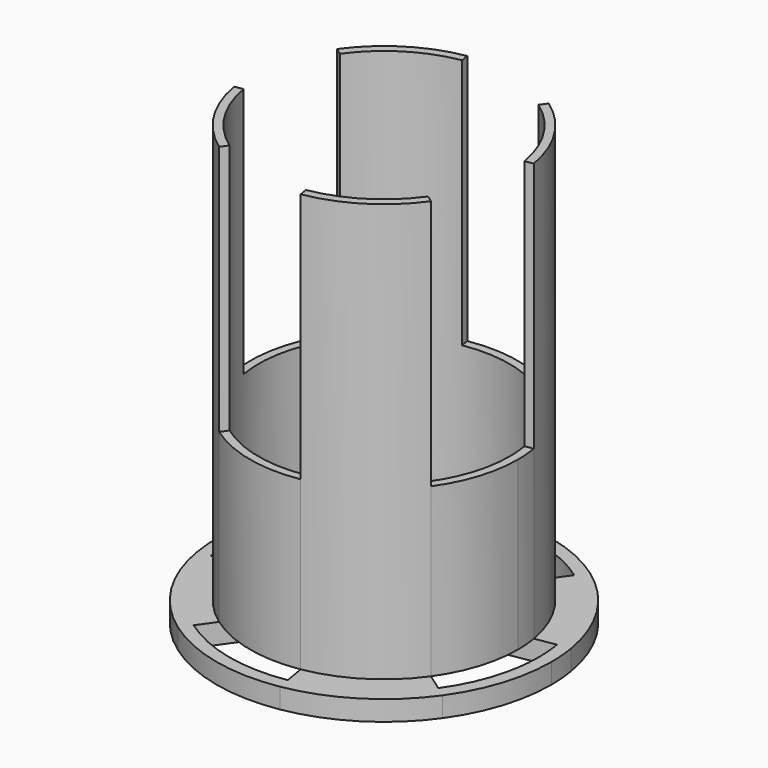
from build123d import *

# Parameters (mm, degrees)
F1_DEPTH = 1.2
F2_DEPTH = 6
F4_DEPTH = 25
F5_DEPTH = 10


with BuildPart() as f1:
    # F0 (on Top) → F1 (new body)
    with BuildSketch(Plane.XY):
        with BuildLine():
            ThreePointArc((8.1482783535, -5.7970302633), (9.5258276159, -3.0427961207), (10, 0))
            ThreePointArc((10, 0), (9.965144828, 0.8341993506), (9.8608222887, 1.6625834689))
            Line((9.8608222887, 1.6625834689), (9.0045502887, -2.0672235383))
            Line((9.0045502887, -2.0672235383), (8.1482783535, -5.7970302633))
        make_face()
        with BuildLine():
            Line((7.8289263433, 4.9054308037), (9.8608222887, 1.6625834689))
            ThreePointArc((9.8608222887, 1.6625834689), (8.4739687378, 5.3096001573), (5.7970302633, 8.1482783535))
            Line((5.7970302633, 8.1482783535), (7.8289263433, 4.9054308037))
        make_face()
        with BuildLine():
            Line((9.1102118863, 1.536026838), (9.8608222887, 1.6625834689))
            Line((9.8608222887, 1.6625834689), (7.8289263433, 4.9054308037))
            ThreePointArc((7.8289263433, 4.9054308037), (8.6354977715, 3.2838266242), (9.1102118863, 1.536026838))
        make_face()
        with BuildLine():
            Line((9.0045502887, -2.0672235383), (9.8608222887, 1.6625834689))
            Line((9.8608222887, 1.6625834689), (9.1102118863, 1.536026838))
            ThreePointArc((9.1102118863, 1.536026838), (9.2065933451, 0.7706997061), (9.2387953251, 0))
            ThreePointArc((9.2387953251, 0), (9.1800472812, -1.040226405), (9.0045502887, -2.0672235383))
        make_face()
        with BuildLine():
            Line((7.528027596, -5.3557576096), (8.1482783535, -5.7970302633))
            Line((8.1482783535, -5.7970302633), (9.0045502887, -2.0672235383))
            ThreePointArc((9.0045502887, -2.0672235383), (8.4282351037, -3.7842029671), (7.528027596, -5.3557576096))
        make_face()
        with BuildLine():
            ThreePointArc((1.6625834689, -9.8608222887), (5.3096001573, -8.4739687378), (8.1482783535, -5.7970302633))
            Line((8.1482783535, -5.7970302633), (4.9054307168, -7.8289263978))
            Line((4.9054307168, -7.8289263978), (1.6625834689, -9.8608222887))
        make_face()
        with BuildLine():
            Line((4.9054307168, -7.8289263978), (8.1482783535, -5.7970302633))
            Line((8.1482783535, -5.7970302633), (7.528027596, -5.3557576096))
            ThreePointArc((7.528027596, -5.3557576096), (6.3385220965, -6.7214936355), (4.9054307168, -7.8289263978))
        make_face()
        with BuildLine():
            Line((2.0672236693, 9.0045502586), (5.7970302633, 8.1482783535))
            ThreePointArc((5.7970302633, 8.1482783535), (2.2375464814, 9.7464550347), (-1.6625834689, 9.8608222887))
            Line((-1.6625834689, 9.8608222887), (2.0672236693, 9.0045502586))
        make_face()
        with BuildLine():
            Line((5.3557576096, 7.528027596), (5.7970302633, 8.1482783535))
            Line((5.7970302633, 8.1482783535), (2.0672236693, 9.0045502586))
            ThreePointArc((2.0672236693, 9.0045502586), (3.7842030284, 8.4282350762), (5.3557576096, 7.528027596))
        make_face()
        with BuildLine():
            Line((7.8289263433, 4.9054308037), (5.7970302633, 8.1482783535))
            Line((5.7970302633, 8.1482783535), (5.3557576096, 7.528027596))
            ThreePointArc((5.3557576096, 7.528027596), (6.7214936003, 6.3385221338), (7.8289263433, 4.9054308037))
        make_face()
        with BuildLine():
            Line((1.536026838, -9.1102118863), (1.6625834689, -9.8608222887))
            Line((1.6625834689, -9.8608222887), (4.9054307168, -7.8289263978))
            ThreePointArc((4.9054307168, -7.8289263978), (3.2838265763, -8.6354977897), (1.536026838, -9.1102118863))
        make_face()
        with BuildLine():
            ThreePointArc((-5.7970302633, -8.1482783535), (-2.2375464814, -9.7464550347), (1.6625834689, -9.8608222887))
            Line((1.6625834689, -9.8608222887), (-2.0672231954, -9.0045503674))
            Line((-2.0672231954, -9.0045503674), (-5.7970302633, -8.1482783535))
        make_face()
        with BuildLine():
            Line((-2.0672231954, -9.0045503674), (1.6625834689, -9.8608222887))
            Line((1.6625834689, -9.8608222887), (1.536026838, -9.1102118863))
            ThreePointArc((1.536026838, -9.1102118863), (-0.2708015541, -9.2348256929), (-2.0672231954, -9.0045503674))
        make_face()
        with BuildLine():
            Line((-4.9054310148, 7.828926211), (-1.6625834689, 9.8608222887))
            ThreePointArc((-1.6625834689, 9.8608222887), (-5.3096001573, 8.4739687378), (-8.1482783535, 5.7970302633))
            Line((-8.1482783535, 5.7970302633), (-4.9054310148, 7.828926211))
        make_face()
        with BuildLine():
            Line((-1.536026838, 9.1102118863), (-1.6625834689, 9.8608222887))
            Line((-1.6625834689, 9.8608222887), (-4.9054310148, 7.828926211))
            ThreePointArc((-4.9054310148, 7.828926211), (-3.2838267407, 8.6354977272), (-1.536026838, 9.1102118863))
        make_face()
        with BuildLine():
            Line((2.0672236693, 9.0045502586), (-1.6625834689, 9.8608222887))
            Line((-1.6625834689, 9.8608222887), (-1.536026838, 9.1102118863))
            ThreePointArc((-1.536026838, 9.1102118863), (0.2708017971, 9.2348256857), (2.0672236693, 9.0045502586))
        make_face()
        with BuildLine():
            Line((-5.3557576096, -7.528027596), (-5.7970302633, -8.1482783535))
            Line((-5.7970302633, -8.1482783535), (-2.0672231954, -9.0045503674))
            ThreePointArc((-2.0672231954, -9.0045503674), (-3.7842028066, -8.4282351757), (-5.3557576096, -7.528027596))
        make_face()
        with BuildLine():
            ThreePointArc((-9.8608222887, -1.6625834689), (-8.4739687378, -5.3096001573), (-5.7970302633, -8.1482783535))
            Line((-5.7970302633, -8.1482783535), (-7.8289263978, -4.9054307168))
            Line((-7.8289263978, -4.9054307168), (-9.8608222887, -1.6625834689))
        make_face()
        with BuildLine():
            Line((-7.8289263978, -4.9054307168), (-5.7970302633, -8.1482783535))
            Line((-5.7970302633, -8.1482783535), (-5.3557576096, -7.528027596))
            ThreePointArc((-5.3557576096, -7.528027596), (-6.7214936355, -6.3385220965), (-7.8289263978, -4.9054307168))
        make_face()
        with BuildLine():
            Line((-9.004550337, 2.0672233281), (-8.1482783535, 5.7970302633))
            ThreePointArc((-8.1482783535, 5.7970302633), (-9.7464550347, 2.2375464814), (-9.8608222887, -1.6625834689))
            Line((-9.8608222887, -1.6625834689), (-9.004550337, 2.0672233281))
        make_face()
        with BuildLine():
            Line((-7.528027596, 5.3557576096), (-8.1482783535, 5.7970302633))
            Line((-8.1482783535, 5.7970302633), (-9.004550337, 2.0672233281))
            ThreePointArc((-9.004550337, 2.0672233281), (-8.4282351479, 3.7842028687), (-7.528027596, 5.3557576096))
        make_face()
        with BuildLine():
            Line((-4.9054310148, 7.828926211), (-8.1482783535, 5.7970302633))
            Line((-8.1482783535, 5.7970302633), (-7.528027596, 5.3557576096))
            ThreePointArc((-7.528027596, 5.3557576096), (-6.3385222244, 6.7214935148), (-4.9054310148, 7.828926211))
        make_face()
        with BuildLine():
            Line((-9.1102118863, -1.536026838), (-9.8608222887, -1.6625834689))
            Line((-9.8608222887, -1.6625834689), (-7.8289263978, -4.9054307168))
            ThreePointArc((-7.8289263978, -4.9054307168), (-8.6354977897, -3.2838265763), (-9.1102118863, -1.536026838))
        make_face()
        with BuildLine():
            Line((-9.004550337, 2.0672233281), (-9.8608222887, -1.6625834689))
            Line((-9.8608222887, -1.6625834689), (-9.1102118863, -1.536026838))
            ThreePointArc((-9.1102118863, -1.536026838), (-9.2348256909, 0.2708016221), (-9.004550337, 2.0672233281))
        make_face()
        with BuildLine():
            ThreePointArc((-4.9304111443, -0.8312917344), (-4.2369843689, -2.6548000787), (-2.8985151316, -4.0741391768))
            Line((-2.8985151316, -4.0741391768), (-1.1594060527, -1.6296556707))
            ThreePointArc((-1.1594060527, -1.6296556707), (-1.6947937476, -1.0619200315), (-1.9721644577, -0.3325166938))
            Line((-1.9721644577, -0.3325166938), (-4.9304111443, -0.8312917344))
        make_face()
        with BuildLine():
            Line((-1.6296556707, 1.1594060527), (-4.0741391768, 2.8985151316))
            ThreePointArc((-4.0741391768, 2.8985151316), (-4.8732275174, 1.1187732407), (-4.9304111443, -0.8312917344))
            Line((-4.9304111443, -0.8312917344), (-1.9721644577, -0.3325166938))
            ThreePointArc((-1.9721644577, -0.3325166938), (-1.9492910069, 0.4475092963), (-1.6296556707, 1.1594060527))
        make_face()
        with BuildLine():
            Line((-0.3325166938, 1.9721644577), (-0.8312917344, 4.9304111443))
            ThreePointArc((-0.8312917344, 4.9304111443), (-2.6548000787, 4.2369843689), (-4.0741391768, 2.8985151316))
            Line((-4.0741391768, 2.8985151316), (-1.6296556707, 1.1594060527))
            ThreePointArc((-1.6296556707, 1.1594060527), (-1.0619200315, 1.6947937476), (-0.3325166938, 1.9721644577))
        make_face()
        with BuildLine():
            Line((1.1594060527, 1.6296556707), (2.8985151316, 4.0741391768))
            ThreePointArc((2.8985151316, 4.0741391768), (1.1187732407, 4.8732275174), (-0.8312917344, 4.9304111443))
            Line((-0.8312917344, 4.9304111443), (-0.3325166938, 1.9721644577))
            ThreePointArc((-0.3325166938, 1.9721644577), (0.4475092963, 1.9492910069), (1.1594060527, 1.6296556707))
        make_face()
        with BuildLine():
            Line((1.9721644577, 0.3325166938), (4.9304111443, 0.8312917344))
            ThreePointArc((4.9304111443, 0.8312917344), (4.2369843689, 2.6548000787), (2.8985151316, 4.0741391768))
            Line((2.8985151316, 4.0741391768), (1.1594060527, 1.6296556707))
            ThreePointArc((1.1594060527, 1.6296556707), (1.6947937476, 1.0619200315), (1.9721644577, 0.3325166938))
        make_face()
        with BuildLine():
            ThreePointArc((5, 0), (4.982572414, 0.4170996753), (4.9304111443, 0.8312917344))
            Line((4.9304111443, 0.8312917344), (1.9721644577, 0.3325166938))
            ThreePointArc((1.9721644577, 0.3325166938), (1.9930289656, 0.1668398701), (2, 0))
            ThreePointArc((2, 0), (1.9051655232, -0.6085592241), (1.6296556707, -1.1594060527))
            Line((1.6296556707, -1.1594060527), (4.0741391768, -2.8985151316))
            ThreePointArc((4.0741391768, -2.8985151316), (4.7629138079, -1.5213980604), (5, 0))
        make_face()
        with BuildLine():
            ThreePointArc((0.8312917344, -4.9304111443), (2.6548000787, -4.2369843689), (4.0741391768, -2.8985151316))
            Line((4.0741391768, -2.8985151316), (1.6296556707, -1.1594060527))
            ThreePointArc((1.6296556707, -1.1594060527), (1.0619200315, -1.6947937476), (0.3325166938, -1.9721644577))
            Line((0.3325166938, -1.9721644577), (0.8312917344, -4.9304111443))
        make_face()
        with BuildLine():
            ThreePointArc((-2.8985151316, -4.0741391768), (-1.1187732407, -4.8732275174), (0.8312917344, -4.9304111443))
            Line((0.8312917344, -4.9304111443), (0.3325166938, -1.9721644577))
            ThreePointArc((0.3325166938, -1.9721644577), (-0.4475092963, -1.9492910069), (-1.1594060527, -1.6296556707))
            Line((-1.1594060527, -1.6296556707), (-2.8985151316, -4.0741391768))
        make_face()
        with BuildLine():
            ThreePointArc((1.536026838, -9.1102118863), (3.2838265763, -8.6354977897), (4.9054307168, -7.8289263978))
            ThreePointArc((4.9054307168, -7.8289263978), (6.3385220965, -6.7214936355), (7.528027596, -5.3557576096))
            Line((7.528027596, -5.3557576096), (4.0741391768, -2.8985151316))
            ThreePointArc((4.0741391768, -2.8985151316), (2.6548000787, -4.2369843689), (0.8312917344, -4.9304111443))
            Line((0.8312917344, -4.9304111443), (1.536026838, -9.1102118863))
        make_face()
        with BuildLine():
            ThreePointArc((9.1102118863, 1.536026838), (8.6354977715, 3.2838266242), (7.8289263433, 4.9054308037))
            ThreePointArc((7.8289263433, 4.9054308037), (6.7214936003, 6.3385221338), (5.3557576096, 7.528027596))
            Line((5.3557576096, 7.528027596), (2.8985151316, 4.0741391768))
            ThreePointArc((2.8985151316, 4.0741391768), (4.2369843689, 2.6548000787), (4.9304111443, 0.8312917344))
            Line((4.9304111443, 0.8312917344), (9.1102118863, 1.536026838))
        make_face()
        with BuildLine():
            ThreePointArc((-1.536026838, 9.1102118863), (-3.2838267407, 8.6354977272), (-4.9054310148, 7.828926211))
            ThreePointArc((-4.9054310148, 7.828926211), (-6.3385222244, 6.7214935148), (-7.528027596, 5.3557576096))
            Line((-7.528027596, 5.3557576096), (-4.0741391768, 2.8985151316))
            ThreePointArc((-4.0741391768, 2.8985151316), (-2.6548000787, 4.2369843689), (-0.8312917344, 4.9304111443))
            Line((-0.8312917344, 4.9304111443), (-1.536026838, 9.1102118863))
        make_face()
        with BuildLine():
            ThreePointArc((-9.1102118863, -1.536026838), (-8.6354977897, -3.2838265763), (-7.8289263978, -4.9054307168))
            ThreePointArc((-7.8289263978, -4.9054307168), (-6.7214936355, -6.3385220965), (-5.3557576096, -7.528027596))
            Line((-5.3557576096, -7.528027596), (-2.8985151316, -4.0741391768))
            ThreePointArc((-2.8985151316, -4.0741391768), (-4.2369843689, -2.6548000787), (-4.9304111443, -0.8312917344))
            Line((-4.9304111443, -0.8312917344), (-9.1102118863, -1.536026838))
        make_face()
    extrude(amount=F1_DEPTH)

    # F0 (on Top) → F2 (join)
    with BuildSketch(Plane.XY):
        with BuildLine():
            Line((-0.1828841816, 1.0846904518), (-0.3325166938, 1.9721644577))
            ThreePointArc((-0.3325166938, 1.9721644577), (-1.0619200315, 1.6947937476), (-1.6296556707, 1.1594060527))
            Line((-1.6296556707, 1.1594060527), (-0.8963106189, 0.637673329))
            ThreePointArc((-0.8963106189, 0.637673329), (-0.5840560173, 0.9321365612), (-0.1828841816, 1.0846904518))
        make_face()
        with BuildLine():
            Line((-0.8963106189, 0.637673329), (-1.6296556707, 1.1594060527))
            ThreePointArc((-1.6296556707, 1.1594060527), (-1.9492910069, 0.4475092963), (-1.9721644577, -0.3325166938))
            Line((-1.9721644577, -0.3325166938), (-1.0846904518, -0.1828841816))
            ThreePointArc((-1.0846904518, -0.1828841816), (-1.0721100538, 0.246130113), (-0.8963106189, 0.637673329))
        make_face()
        with BuildLine():
            ThreePointArc((-1.9721644577, -0.3325166938), (-1.6947937476, -1.0619200315), (-1.1594060527, -1.6296556707))
            Line((-1.1594060527, -1.6296556707), (-0.637673329, -0.8963106189))
            ThreePointArc((-0.637673329, -0.8963106189), (-0.9321365612, -0.5840560173), (-1.0846904518, -0.1828841816))
            Line((-1.0846904518, -0.1828841816), (-1.9721644577, -0.3325166938))
        make_face()
        with BuildLine():
            ThreePointArc((-1.1594060527, -1.6296556707), (-0.4475092963, -1.9492910069), (0.3325166938, -1.9721644577))
            Line((0.3325166938, -1.9721644577), (0.1828841816, -1.0846904518))
            ThreePointArc((0.1828841816, -1.0846904518), (-0.246130113, -1.0721100538), (-0.637673329, -0.8963106189))
            Line((-0.637673329, -0.8963106189), (-1.1594060527, -1.6296556707))
        make_face()
        with BuildLine():
            ThreePointArc((0.3325166938, -1.9721644577), (1.0619200315, -1.6947937476), (1.6296556707, -1.1594060527))
            Line((1.6296556707, -1.1594060527), (0.8963106189, -0.637673329))
            ThreePointArc((0.8963106189, -0.637673329), (0.5840560173, -0.9321365612), (0.1828841816, -1.0846904518))
            Line((0.1828841816, -1.0846904518), (0.3325166938, -1.9721644577))
        make_face()
        with BuildLine():
            ThreePointArc((2, 0), (1.9930289656, 0.1668398701), (1.9721644577, 0.3325166938))
            Line((1.9721644577, 0.3325166938), (1.0846904518, 0.1828841816))
            ThreePointArc((1.0846904518, 0.1828841816), (1.0961659311, 0.0917619286), (1.1, 0))
            ThreePointArc((1.1, 0), (1.0478410377, -0.3347075733), (0.8963106189, -0.637673329))
            Line((0.8963106189, -0.637673329), (1.6296556707, -1.1594060527))
            ThreePointArc((1.6296556707, -1.1594060527), (1.9051655232, -0.6085592241), (2, 0))
        make_face()
        with BuildLine():
            Line((1.0846904518, 0.1828841816), (1.9721644577, 0.3325166938))
            ThreePointArc((1.9721644577, 0.3325166938), (1.6947937476, 1.0619200315), (1.1594060527, 1.6296556707))
            Line((1.1594060527, 1.6296556707), (0.637673329, 0.8963106189))
            ThreePointArc((0.637673329, 0.8963106189), (0.9321365612, 0.5840560173), (1.0846904518, 0.1828841816))
        make_face()
        with BuildLine():
            Line((0.637673329, 0.8963106189), (1.1594060527, 1.6296556707))
            ThreePointArc((1.1594060527, 1.6296556707), (0.4475092963, 1.9492910069), (-0.3325166938, 1.9721644577))
            Line((-0.3325166938, 1.9721644577), (-0.1828841816, 1.0846904518))
            ThreePointArc((-0.1828841816, 1.0846904518), (0.246130113, 1.0721100538), (0.637673329, 0.8963106189))
        make_face()
    extrude(amount=F2_DEPTH)


with BuildPart() as f4:
    # F3 (on face) → F4 (new body)
    with BuildSketch(Plane.XY.offset(1.2)):
        with BuildLine():
            Line((6.5186226828, -4.6376242106), (6.1112087651, -4.3477726975))
            ThreePointArc((6.1112087651, -4.3477726975), (3.982200118, -6.3554765533), (1.2469376016, -7.3956167165))
            Line((1.2469376016, -7.3956167165), (1.3300667751, -7.888657831))
            ThreePointArc((1.3300667751, -7.888657831), (4.2476801259, -6.7791749902), (6.5186226828, -4.6376242106))
        make_face()
    extrude(amount=F4_DEPTH)



with BuildPart() as f4b:
    # F3 (on face) → F4, piece 2 (new body)
    with BuildSketch(Plane.XY.offset(1.2)):
        with BuildLine():
            ThreePointArc((-6.1112087651, 4.3477726975), (-3.982200118, 6.3554765533), (-1.2469376016, 7.3956167165))
            Line((-1.2469376016, 7.3956167165), (-1.3300667751, 7.888657831))
            ThreePointArc((-1.3300667751, 7.888657831), (-4.2476801259, 6.7791749902), (-6.5186226828, 4.6376242106))
            Line((-6.5186226828, 4.6376242106), (-6.1112087651, 4.3477726975))
        make_face()
    extrude(amount=F4_DEPTH)


with BuildPart() as f4c:
    # F3 (on face) → F4, piece 3 (new body)
    with BuildSketch(Plane.XY.offset(1.2)):
        with BuildLine():
            ThreePointArc((4.3477726975, 6.1112087651), (6.3554765533, 3.982200118), (7.3956167165, 1.2469376016))
            Line((7.3956167165, 1.2469376016), (7.888657831, 1.3300667751))
            ThreePointArc((7.888657831, 1.3300667751), (6.7791749902, 4.2476801259), (4.6376242106, 6.5186226828))
            Line((4.6376242106, 6.5186226828), (4.3477726975, 6.1112087651))
        make_face()
    extrude(amount=F4_DEPTH)


with BuildPart() as f4d:
    # F3 (on face) → F4, piece 4 (new body)
    with BuildSketch(Plane.XY.offset(1.2)):
        with BuildLine():
            Line((-4.6376242106, -6.5186226828), (-4.3477726975, -6.1112087651))
            ThreePointArc((-4.3477726975, -6.1112087651), (-6.3554765533, -3.982200118), (-7.3956167165, -1.2469376016))
            Line((-7.3956167165, -1.2469376016), (-7.888657831, -1.3300667751))
            ThreePointArc((-7.888657831, -1.3300667751), (-6.7791749902, -4.2476801259), (-4.6376242106, -6.5186226828))
        make_face()
    extrude(amount=F4_DEPTH)


with BuildPart() as f4_1:
    add(f4.part)

    add(f4b.part)  # F5 merges F4b

    add(f4c.part)  # F5 merges F4c

    add(f4d.part)  # F5 merges F4d
    # F3 (on face) → F5 (join)
    with BuildSketch(Plane.XY.offset(1.2)):
        with BuildLine():
            Line((1.3300667751, -7.888657831), (1.2469376016, -7.3956167165))
            ThreePointArc((1.2469376016, -7.3956167165), (-1.6781598611, -7.309841276), (-4.3477726975, -6.1112087651))
            Line((-4.3477726975, -6.1112087651), (-4.6376242106, -6.5186226828))
            ThreePointArc((-4.6376242106, -6.5186226828), (-1.7900371851, -7.7971640278), (1.3300667751, -7.888657831))
        make_face()
        with BuildLine():
            ThreePointArc((7.3956167165, 1.2469376016), (7.473858621, 0.625649513), (7.5, 0))
            ThreePointArc((7.5, 0), (7.1443707119, -2.2820970906), (6.1112087651, -4.3477726975))
            Line((6.1112087651, -4.3477726975), (6.5186226828, -4.6376242106))
            ThreePointArc((6.5186226828, -4.6376242106), (7.6206620927, -2.4342368966), (8, 0))
            ThreePointArc((8, 0), (7.9721158624, 0.6673594805), (7.888657831, 1.3300667751))
            Line((7.888657831, 1.3300667751), (7.3956167165, 1.2469376016))
        make_face()
        with BuildLine():
            ThreePointArc((-1.2469376016, 7.3956167165), (1.6781598611, 7.309841276), (4.3477726975, 6.1112087651))
            Line((4.3477726975, 6.1112087651), (4.6376242106, 6.5186226828))
            ThreePointArc((4.6376242106, 6.5186226828), (1.7900371851, 7.7971640278), (-1.3300667751, 7.888657831))
            Line((-1.3300667751, 7.888657831), (-1.2469376016, 7.3956167165))
        make_face()
        with BuildLine():
            ThreePointArc((-7.3956167165, -1.2469376016), (-7.309841276, 1.6781598611), (-6.1112087651, 4.3477726975))
            Line((-6.1112087651, 4.3477726975), (-6.5186226828, 4.6376242106))
            ThreePointArc((-6.5186226828, 4.6376242106), (-7.7971640278, 1.7900371851), (-7.888657831, -1.3300667751))
            Line((-7.888657831, -1.3300667751), (-7.3956167165, -1.2469376016))
        make_face()
    extrude(amount=F5_DEPTH)


solid = Compound([f1.part, f4_1.part])
